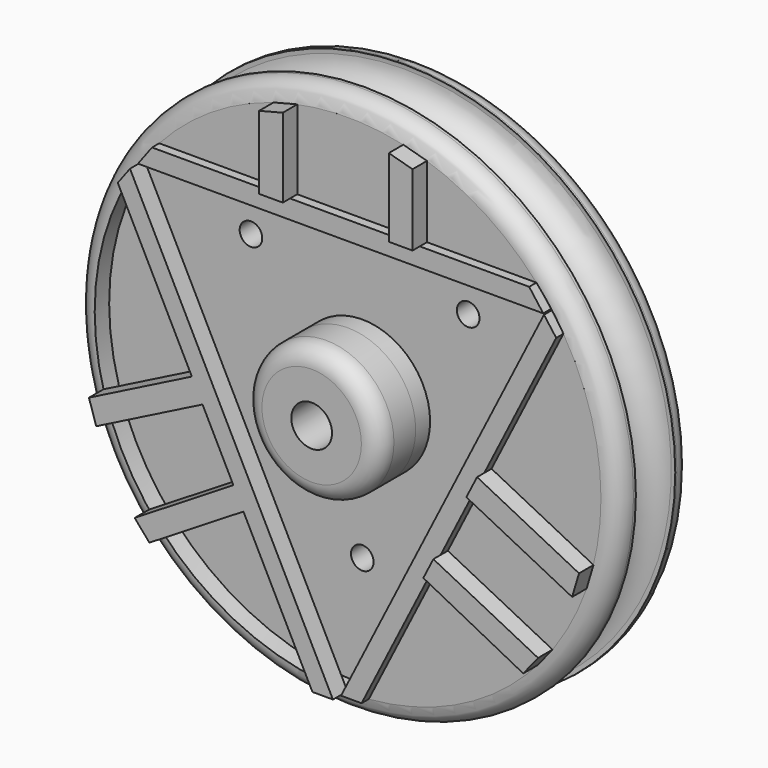
from build123d import *

# Parameters (mm, degrees)
F0_R      = 76.2
F1_DEPTH  = 25.4
F2_R      = 19.05
F3_DEPTH  = 12.7
F4_R      = 5.08
F5_R      = 5.715
F6_DEPTH  = 76.2
F7_R      = 5.08
F8_R      = 7.0297777753
F11_D     = 6.35
F13_DEPTH = 2.54
F14_DEPTH = 5.08
F17_DEPTH = 5.08


# Not quite as in the source:
# - a feature names something its author has since deleted; it is built from what else it names
# - the program builds the solid bodies; features that only make, move or delete a surface that nothing else refers to are left out


with BuildPart() as f1:
    # F0 (on Front) → F1 (new body)
    with BuildSketch(Plane.XZ):
        Circle(F0_R)
    extrude(amount=F1_DEPTH)

    # F2 (on face) → F3 (join)
    with BuildSketch(Plane.XZ.offset(25.4)):
        Circle(F2_R)
    extrude(amount=F3_DEPTH)

    # F4
    f4_edges = [f1.edges().sort_by_distance(p)[0] for p in [
        (-76.2, -25.4, 0),
        (-76.2, 0, 0),
    ]]
    fillet(f4_edges, radius=F4_R)

    # F5 (on face) → F6 (cut)
    with BuildSketch(Plane.XZ.offset(38.1)):
        Circle(F5_R)
    extrude(amount=-F6_DEPTH, mode=Mode.SUBTRACT)

    # F7
    f7_edges = [f1.edges().sort_by_distance(p)[0] for p in [
        (-19.05, -38.1, 0),
    ]]
    fillet(f7_edges, radius=F7_R)

    # F8 (on Right) → F9 (revolve, cut)
    with BuildSketch(Plane.YZ):
        with Locations((-12.5752454624, 74.9799013138)):
            Circle(F8_R)
    revolve(axis=Axis((0, 0, 0), (0, 1, 0)), mode=Mode.SUBTRACT)

    # F11 (through all)
    with Locations(Plane.XZ.offset(25.4)):
        with Locations((-31.2809236348, 29.9864178827), (0, -39.9264059961), (29.7482135823, 29.9864178827)):
            Hole(F11_D / 2)

    # F12 (on face) → F13 (join)
    with BuildSketch(Plane.XZ.offset(25.4)):
        Polygon((60.5736467116, 37.2677839972), (57.137273224, 41.8741591157), (0.1235082642, -70.8757511643), (5.8891677589, -70.8757511643), (25.271153487, -32.5461100077), (28.0907682056, -26.9700652268), (37.3634036013, -8.6325846262), (40.3664078951, -2.693870266), align=None)
        Polygon((-52.9815390901, 47.4448196924), (-56.9276816511, 42.155660184), (56.9272723486, 42.155660184), (52.9815390901, 47.4448196924), (22.2352999541, 47.4448196924), (15.5804999541, 47.4448196924), (-14.2111172058, 47.4448196924), (-20.8659172058, 47.4448196924), align=None)
    extrude(amount=F13_DEPTH)

    # F17 (cut): a face of the model
    f17_faces = [f1.faces().sort_by_distance(p)[0] for p in [
        (58.9974941885, -25.4, 39.6769296293),
    ]]
    extrude(f17_faces, amount=-F17_DEPTH, mode=Mode.SUBTRACT)


with BuildPart() as f14:
    # F12 (on face) → F14 (new body)
    with BuildSketch(Plane.XZ.offset(25.4)):
        Polygon((-0.1235082642, -70.8757511643), (-57.1374473692, 41.8745035037), (-60.5699408845, 37.2738066374), (-39.7584415253, -3.8879093412), (-36.761269241, -9.8158221829), (-28.0937840544, -26.9586794726), (-25.2646825431, -32.5541760235), (-5.8891677589, -70.8757511643), align=None)
        Polygon((-36.761269241, -9.8158221829), (-39.7584415253, -3.8879093412), (-68.6701601192, -18.5057696195), (-66.6149351284, -24.9099341196), align=None)
        Polygon((-51.6881021847, -48.850736868), (-25.2646825431, -32.5541760235), (-28.0937840544, -26.9586794726), (-55.8260833114, -44.0624876976), align=None)
    extrude(amount=F14_DEPTH)


with BuildPart() as f14b:
    # F12 (on face) → F14, piece 2 (new body)
    with BuildSketch(Plane.XZ.offset(25.4)):
        Polygon((28.0907682056, -26.9700652268), (25.271153487, -32.5461100077), (53.3431713755, -47.0378620646), (57.5070525493, -41.8448719331), align=None)
    extrude(amount=F14_DEPTH)


with BuildPart() as f14c:
    # F12 (on face) → F14, piece 3 (new body)
    with BuildSketch(Plane.XZ.offset(25.4)):
        Polygon((69.0138110743, -17.1798801219), (40.3664078951, -2.693870266), (37.3634036013, -8.6325846262), (67.0709407107, -23.6546678729), align=None)
    extrude(amount=F14_DEPTH)


with BuildPart() as f14d:
    # F12 (on face) → F14, piece 4 (new body)
    with BuildSketch(Plane.XZ.offset(25.4)):
        Polygon((15.5804999541, 47.4448196924), (22.2352999541, 47.4448196924), (22.2352999541, 67.5547617563), (15.5804999541, 69.3923801377), align=None)
    extrude(amount=F14_DEPTH)


with BuildPart() as f14e:
    # F12 (on face) → F14, piece 5 (new body)
    with BuildSketch(Plane.XZ.offset(25.4)):
        Polygon((-20.8659172058, 67.9902044353), (-20.8659172058, 47.4448196924), (-14.2111172058, 47.4448196924), (-14.2111172058, 69.6857126516), align=None)
    extrude(amount=F14_DEPTH)


solid = Compound([f1.part, f14.part, f14b.part, f14c.part, f14d.part, f14e.part])
